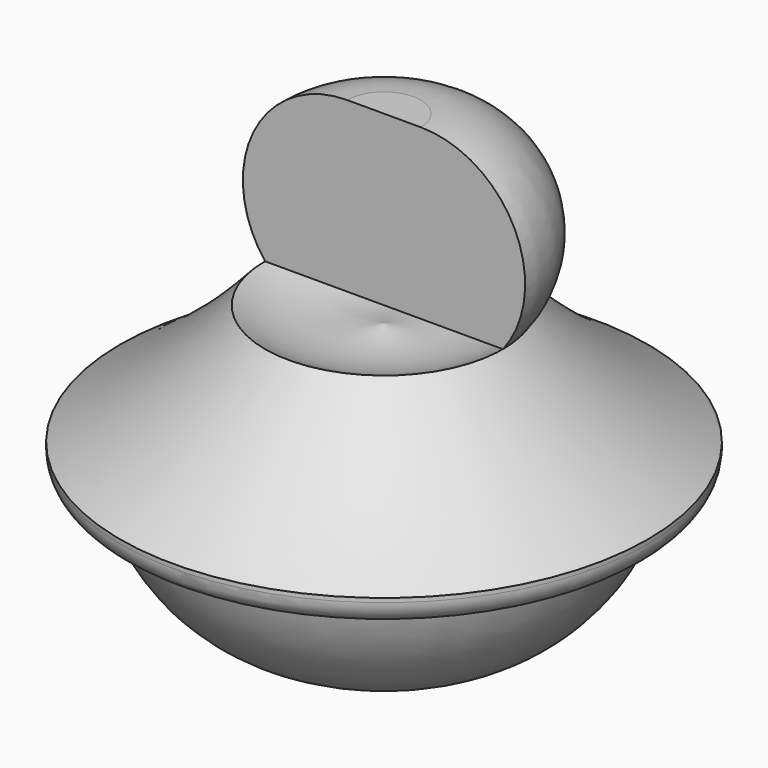
from build123d import *

# Parameters (mm, degrees)
F2_R     = 1.27
F5_W     = 28.0556213111
F5_H     = 15.8260483295
F6_DEPTH = 25.4


with BuildPart() as f1:
    # F0 (on Front) → F1 (revolve)
    with BuildSketch(Plane.XZ):
        with BuildLine():
            ThreePointArc((-11.905984953, 7.4474178255), (-7.5556070937, 1.1616523766), (0, 0))
            Line((0, 0), (0, 7.4474178255))
            Line((0, 7.4474178255), (-11.905984953, 7.4474178255))
        make_face()
        with BuildLine():
            Line((-11.905984953, 7.4474178255), (0, 7.4474178255))
            Line((0, 7.4474178255), (0, 14.5316230621))
            ThreePointArc((0, 14.5316230621), (-3.2714384324, 14.29073486), (-6.3665207505, 15.3773819909))
            ThreePointArc((-6.3665207505, 15.3773819909), (-10.0104927669, 11.8772257791), (-14.119816944, 8.9373141527))
            Line((-14.119816944, 8.9373141527), (-14.119816944, 7.4474178255))
            Line((-14.119816944, 7.4474178255), (-11.905984953, 7.4474178255))
        make_face()
    revolve(axis=Axis((0, 0, 34.3446284533), (0, 0, 1)))

    # F2
    f2_edges = [f1.edges().sort_by_distance(p)[0] for p in [
        (14.119817, 0, 7.447418),
    ]]
    fillet(f2_edges, radius=F2_R)


with BuildPart() as f4:
    # F3 (on Front) → F4 (revolve)
    with BuildSketch(Plane.XZ):
        with BuildLine():
            Line((-6.3665207505, 15.3773819909), (0, 15.3773819909))
            Line((0, 15.3773819909), (0, 24.4007859645))
            Line((0, 24.4007859645), (-1.9672751456, 24.4007859645))
            ThreePointArc((-1.9672751456, 24.4007859645), (-6.986617263, 21.2638021926), (-6.3665207505, 15.3773819909))
        make_face()
    revolve(axis=Axis((0, 0, 22.8794236608), (0, 0, 1)))

    # F5 (on Front) → F6 (cut)
    with BuildSketch(Plane.XZ):
        with Locations((1.4464305714, 21.0229521617)):
            Rectangle(F5_W, F5_H)
    extrude(amount=F6_DEPTH, mode=Mode.SUBTRACT)


solid = Compound([f1.part, f4.part])
